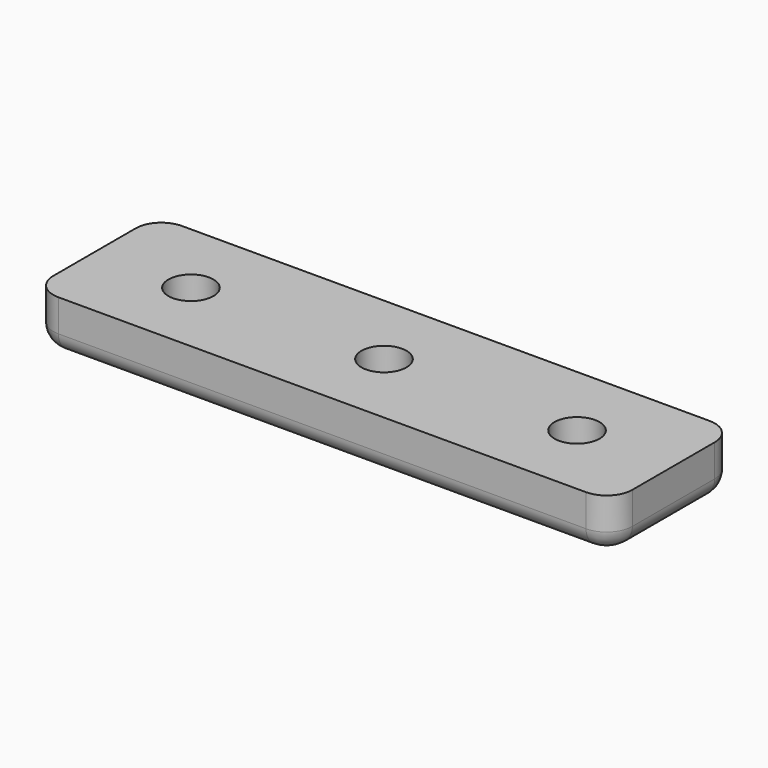
from build123d import *

# Parameters (mm, degrees)
F0_W           = 45
F0_H           = 12
F1_DEPTH       = 4
F2_D           = 3.5
F2_CSINK_D     = 5
F2_CSINK_ANGLE = 90
F3_R           = 1.5
F4_T1_DEPTH    = 9
F4_T4_ANGLE    = 90
F4_T6_ANGLE    = 90
F4_T8_ANGLE    = 90
F4_T10_ANGLE   = 90


# Not quite as in the source:
# - a fillet or chamfer that OpenCascade refuses, or shapes differently, is made with other operations: its cross-section is extruded or revolved along the edge and cut away or added


with BuildPart() as f1:
    # F0 (on Top) → F1 (new body)
    with BuildSketch(Plane.XY):
        Rectangle(F0_W, F0_H)
    extrude(amount=F1_DEPTH)

    # F2 (through all)
    with Locations(Plane(origin=(0, 0, 0), x_dir=(1, 0, 0), z_dir=(0, 0, -1))):
        with Locations((-15, 0), (0, 0), (15, 0)):
            CounterSinkHole(F2_D / 2, F2_CSINK_D / 2, counter_sink_angle=F2_CSINK_ANGLE)

    # F3
    f3_edges = [f1.edges().sort_by_distance(p)[0] for p in [
        (0, -6, 0),
        (-22.5, 0, 0),
        (0, 6, 0),
        (22.5, 0, 0),
    ]]
    fillet(f3_edges, radius=F3_R)

    # F4: fillet of radius 2 on 4 edges, made by hand

    # F4_s2 → F4_t1 (cut)
    with BuildSketch(Plane.XY):
        with BuildLine():
            ThreePointArc((22.5, -4), (21.9142135624, -5.4142135624), (20.5, -6))
            Line((20.5, -6), (22.5, -6))
            Line((22.5, -6), (22.5, -4))
        make_face()
        with BuildLine():
            ThreePointArc((20.5, 6), (21.9142135624, 5.4142135624), (22.5, 4))
            Line((22.5, 4), (22.5, 6))
            Line((22.5, 6), (20.5, 6))
        make_face()
        with BuildLine():
            ThreePointArc((-22.5, -4), (-21.9142135624, -5.4142135624), (-20.5, -6))
            Line((-20.5, -6), (-22.5, -6))
            Line((-22.5, -6), (-22.5, -4))
        make_face()
        with BuildLine():
            ThreePointArc((-20.5, 6), (-21.9142135624, 5.4142135624), (-22.5, 4))
            Line((-22.5, 4), (-22.5, 6))
            Line((-22.5, 6), (-20.5, 6))
        make_face()
    extrude(amount=F4_T1_DEPTH, mode=Mode.SUBTRACT)

    # F4_s3 → F4_t4 (revolve, cut)
    with BuildSketch(Plane.XZ.offset(-4)):
        with BuildLine():
            ThreePointArc((-21, 0), (-22.0606601718, 0.4393398282), (-22.5, 1.5))
            Line((-22.5, 1.5), (-22.5, 0))
            Line((-22.5, 0), (-21, 0))
        make_face()
    revolve(axis=Axis((-20.5, 4, 0), (0, 0, -1)), revolution_arc=F4_T4_ANGLE, mode=Mode.SUBTRACT)

    # F4_s5 → F4_t6 (revolve, cut)
    with BuildSketch(Plane.YZ.offset(-20.5)):
        with BuildLine():
            ThreePointArc((-4.5, 0), (-5.5606601718, 0.4393398282), (-6, 1.5))
            Line((-6, 1.5), (-6, 0))
            Line((-6, 0), (-4.5, 0))
        make_face()
    revolve(axis=Axis((-20.5, -4, 0), (0, 0, -1)), revolution_arc=F4_T6_ANGLE, mode=Mode.SUBTRACT)

    # F4_s7 → F4_t8 (revolve, cut)
    with BuildSketch(Plane.YZ.offset(20.5)):
        with BuildLine():
            ThreePointArc((4.5, 0), (5.5606601718, 0.4393398282), (6, 1.5))
            Line((6, 1.5), (6, 0))
            Line((6, 0), (4.5, 0))
        make_face()
    revolve(axis=Axis((20.5, 4, 0), (0, 0, -1)), revolution_arc=F4_T8_ANGLE, mode=Mode.SUBTRACT)

    # F4_s9 → F4_t10 (revolve, cut)
    with BuildSketch(Plane.XZ.offset(4)):
        with BuildLine():
            ThreePointArc((21, 0), (22.0606601718, 0.4393398282), (22.5, 1.5))
            Line((22.5, 1.5), (22.5, 0))
            Line((22.5, 0), (21, 0))
        make_face()
    revolve(axis=Axis((20.5, -4, 0), (0, 0, -1)), revolution_arc=F4_T10_ANGLE, mode=Mode.SUBTRACT)


solid = f1.part
